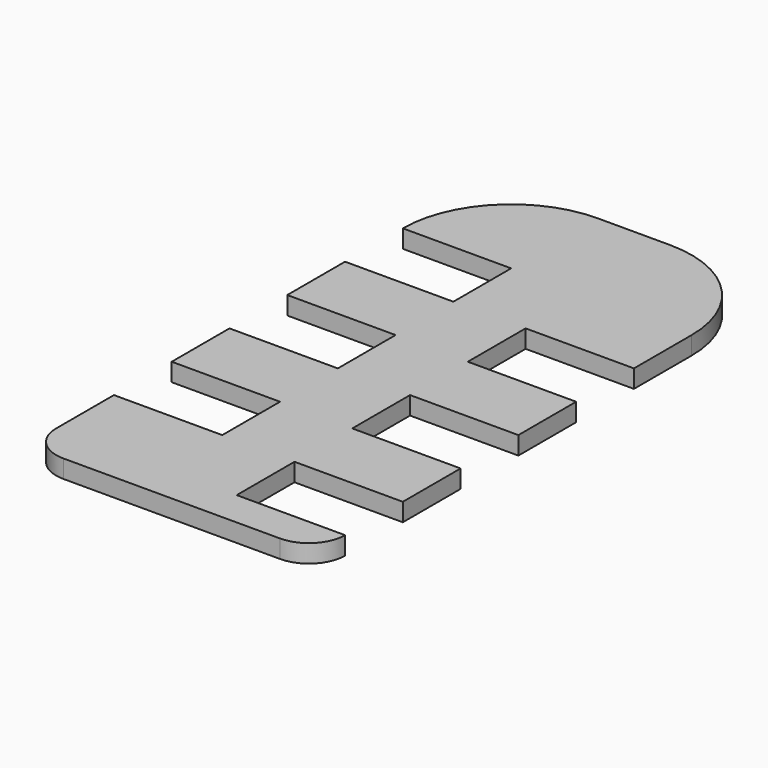
from build123d import *

# Parameters (mm, degrees)
F0_W     = 19.05
F0_H     = 12.694532901
F0_H_2   = 12.7
F1_DEPTH = 3.175


# Not quite as in the source:
# - a length typed as a fraction of an inch, garbled in the dataset ("3 / 203.2 mm" for 3/8 in), is restored


with BuildPart() as f1:
    # F0 (on Top) → F1 (new body)
    with BuildSketch(Plane.XY):
        with BuildLine():
            Line((6.35, 50.8), (-6.35, 50.8))
            ThreePointArc((-6.35, 50.8), (-19.8203841816, 45.2203841816), (-25.4, 31.75))
            Line((-25.4, 31.75), (-6.35, 31.75))
            Line((-6.35, 31.75), (6.35, 31.75))
            Line((6.35, 31.75), (25.4, 31.75))
            ThreePointArc((25.4, 31.75), (19.8203841816, 45.2203841816), (6.35, 50.8))
        make_face()
        with BuildLine():
            Line((6.35, 31.75), (-6.35, 31.75))
            Line((-6.35, 31.75), (-6.35, 19.05))
            Line((-6.35, 19.05), (-6.35, 6.35))
            Line((-6.35, 6.35), (-6.35, -6.35))
            Line((-6.35, -6.35), (-6.35, -19.05))
            Line((-6.35, -19.05), (-6.35, -31.75))
            Line((-6.35, -31.75), (-25.4, -31.75))
            Line((-25.4, -31.75), (-25.4, -44.45))
            ThreePointArc((-25.4, -44.45), (-23.5401280605, -48.9401280605), (-19.05, -50.8))
            Line((-19.05, -50.8), (19.05, -50.8))
            ThreePointArc((19.05, -50.8), (23.5401280605, -48.9401280605), (25.4, -44.45))
            Line((25.4, -44.45), (6.35, -44.45))
            Line((6.35, -44.45), (6.35, -31.75))
            Line((6.35, -31.75), (6.35, -19.05))
            Line((6.35, -19.05), (6.35, -6.35))
            Line((6.35, -6.35), (6.35, 6.35))
            Line((6.35, 6.35), (6.35, 19.055467099))
            Line((6.35, 19.055467099), (6.35, 31.75))
        make_face()
        with Locations((15.875, 25.4027335495)):
            Rectangle(F0_W, F0_H)
        with Locations((15.875, 0)):
            Rectangle(F0_W, F0_H_2)
        with Locations((15.875, -25.4)):
            Rectangle(F0_W, F0_H_2)
        with Locations((-15.875, -12.7)):
            Rectangle(F0_W, F0_H_2)
        with Locations((-15.875, 12.7)):
            Rectangle(F0_W, F0_H_2)
    extrude(amount=F1_DEPTH)


with BuildPart() as f2_1:
    # F2: copy of F1
    add(f1.part)


solid = Compound([f1.part, f2_1.part])
